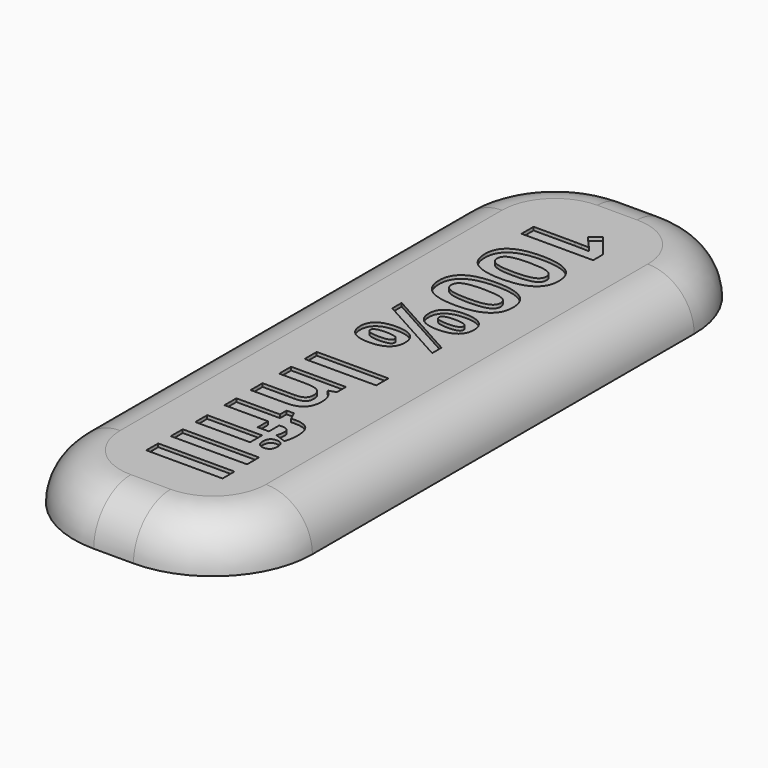
from build123d import *

# Parameters (mm, degrees)
F0_W         = 36
F0_H         = 102
F1_DEPTH     = 3.5
F2_R         = 15
F3_R         = 6.99999
F4_TEXT_SIZE = 15.1433338389
F5_DEPTH     = 0.5


# Not quite as in the source:
# - a fillet or chamfer is up to 0.001 mm smaller than in the source, because OpenCascade refuses the exact size
# - Text() gives the source's letters only with a copy of the font that has no kerning and outlines rounded to 1/6400 em; it was checked with that copy


with BuildPart() as f1:
    # F0 (on Top) → F1 (new body, symmetric)
    with BuildSketch(Plane.XY):
        Rectangle(F0_W, F0_H)
    extrude(amount=F1_DEPTH, both=True)

    # F2
    f2_edges = [f1.edges().sort_by_distance(p)[0] for p in [
        (-18, -51, 0),
        (18, -51, 0),
        (18, 51, 0),
        (-18, 51, 0),
    ]]
    fillet(f2_edges, radius=F2_R)

    # F3 (radius 7 in the source; OpenCascade refuses exactly that, so slightly less here)
    f3_edges = [f1.edges().sort_by_distance(p)[0] for p in [
        (0, -51, 3.5),
        (-13.606602, -46.606602, 3.5),
        (13.606602, -46.606602, 3.5),
        (-18, 0, 3.5),
        (18, 0, 3.5),
        (-13.606602, 46.606602, 3.5),
        (13.606602, 46.606602, 3.5),
        (0, 51, 3.5),
    ]]
    fillet(f3_edges, radius=F3_R)

    # F4 (on face) → F5 (cut)
    with BuildSketch(Plane.XY.offset(3.5)):
        with Locations(Location((-5.451600182, 39), (0, 0, -90))):
            Text('100% Infill', F4_TEXT_SIZE, font='Open Sans', font_style=FontStyle.BOLD, text_align=(TextAlign.LEFT, TextAlign.BOTTOM))
    extrude(amount=-F5_DEPTH, mode=Mode.SUBTRACT)


solid = f1.part
